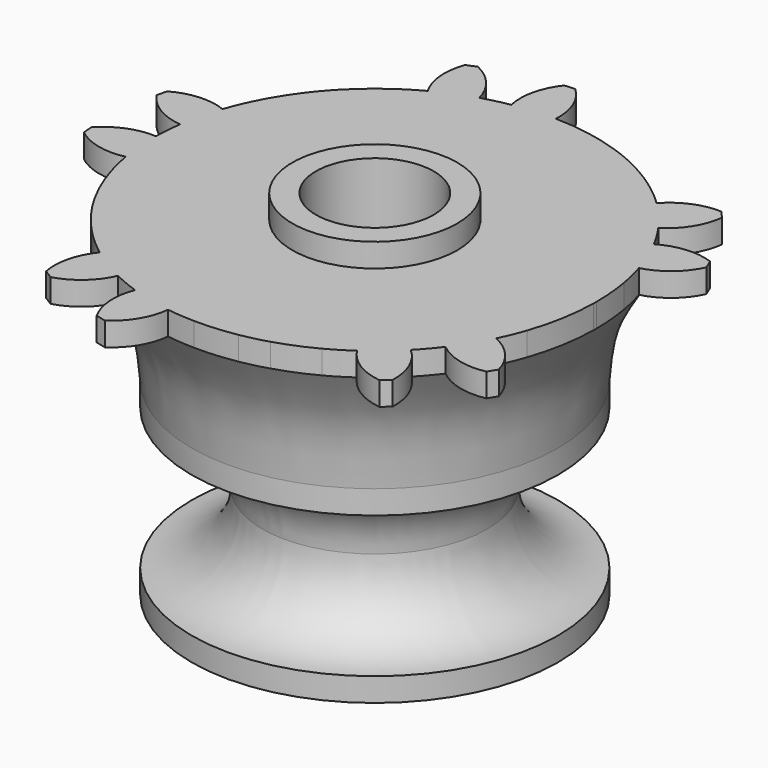
from build123d import *

# Parameters (mm, degrees)
F1_R      = 3.5
F1_R_2    = 2.5
F2_DEPTH  = 1
F3_DEPTH  = 2
F5_R      = 4.7747891135
F5_R_2    = 2.5
F6_DEPTH  = 6
F5_R_3    = 7.7747891135
F7_DEPTH  = 1
F8_DEPTH  = 6
F9_R      = 7.7747891135
F9_R_2    = 4.7747891135
F9_R_3    = 2.5
F10_DEPTH = 1


# Not quite as in the source:
# - a feature names something its author has since deleted; it is built from what else it names


with BuildPart() as f2:
    # F1 (on Top) → F2 (new body)
    with BuildSketch(Plane.XY):
        with BuildLine():
            ThreePointArc((-1.6229776334, 9.2680599554), (-0.7382287643, 9.3800858219), (0.1531520845, 9.4078443957))
            ThreePointArc((0.1531520845, 9.4078443957), (-0.0317997207, 10.5374998224), (-0.6817601701, 11.4797736507))
            Line((-0.6817601701, 11.4797736507), (-1.1224656787, 11.4450893749))
            ThreePointArc((-1.1224656787, 11.4450893749), (-1.6170199342, 10.4127402859), (-1.6229776334, 9.2680599554))
        make_face()
        with BuildLine():
            ThreePointArc((9.4078443957, -0.1531520845), (9.4087792756, -0.0765785786), (9.4090909091, 0))
            ThreePointArc((9.4090909091, 0), (9.3737668631, 0.8145468262), (9.2680599554, 1.6229776334))
            ThreePointArc((9.2680599554, 1.6229776334), (9.1491169783, 2.1965086508), (8.9947183137, 2.7615275108))
            ThreePointArc((8.9947183137, 2.7615275108), (8.6928665104, 3.6007032045), (8.3129211438, 4.4075314852))
            ThreePointArc((8.3129211438, 4.4075314852), (8.0225688191, 4.9162364953), (7.7011265332, 5.4058895526))
            ThreePointArc((7.7011265332, 5.4058895526), (7.1547288581, 6.1107157275), (6.5440556911, 6.7606454461))
            ThreePointArc((6.5440556911, 6.7606454461), (6.1107157275, 7.1547288581), (5.6536948308, 7.52108546))
            ThreePointArc((5.6536948308, 7.52108546), (4.9162364953, 8.0225688191), (4.1346124722, 8.4519803265))
            ThreePointArc((4.1346124722, 8.4519803265), (3.6007032045, 8.6928665104), (3.0528400867, 8.90006512))
            ThreePointArc((3.0528400867, 8.90006512), (2.1965086508, 9.1491169783), (1.320444577, 9.3159764842))
            ThreePointArc((1.320444577, 9.3159764842), (0.7382287643, 9.3800858219), (0.1531520845, 9.4078443957))
            ThreePointArc((0.1531520845, 9.4078443957), (-0.7382287643, 9.3800858219), (-1.6229776334, 9.2680599554))
            ThreePointArc((-1.6229776334, 9.2680599554), (-2.1965086508, 9.1491169783), (-2.7615275108, 8.9947183137))
            ThreePointArc((-2.7615275108, 8.9947183137), (-3.6007032045, 8.6928665104), (-4.4075314852, 8.3129211438))
            ThreePointArc((-4.4075314852, 8.3129211438), (-4.9162364953, 8.0225688191), (-5.4058895526, 7.7011265332))
            ThreePointArc((-5.4058895526, 7.7011265332), (-6.1107157275, 7.1547288581), (-6.7606454461, 6.5440556911))
            ThreePointArc((-6.7606454461, 6.5440556911), (-7.1547288581, 6.1107157275), (-7.52108546, 5.6536948308))
            ThreePointArc((-7.52108546, 5.6536948308), (-8.0225688191, 4.9162364953), (-8.4519803265, 4.1346124722))
            ThreePointArc((-8.4519803265, 4.1346124722), (-8.6928665104, 3.6007032045), (-8.90006512, 3.0528400867))
            ThreePointArc((-8.90006512, 3.0528400867), (-9.1491169783, 2.1965086508), (-9.3159764842, 1.320444577))
            ThreePointArc((-9.3159764842, 1.320444577), (-9.3800858219, 0.7382287643), (-9.4078443957, 0.1531520845))
            ThreePointArc((-9.4078443957, 0.1531520845), (-9.3800858219, -0.7382287643), (-9.2680599554, -1.6229776334))
            ThreePointArc((-9.2680599554, -1.6229776334), (-9.1491169783, -2.1965086508), (-8.9947183137, -2.7615275108))
            ThreePointArc((-8.9947183137, -2.7615275108), (-8.6928665104, -3.6007032045), (-8.3129211438, -4.4075314852))
            ThreePointArc((-8.3129211438, -4.4075314852), (-8.0225688191, -4.9162364953), (-7.7011265332, -5.4058895526))
            ThreePointArc((-7.7011265332, -5.4058895526), (-7.1547288581, -6.1107157275), (-6.5440556911, -6.7606454461))
            ThreePointArc((-6.5440556911, -6.7606454461), (-6.1107157275, -7.1547288581), (-5.6536948308, -7.52108546))
            ThreePointArc((-5.6536948308, -7.52108546), (-4.9162364953, -8.0225688191), (-4.1346124722, -8.4519803265))
            ThreePointArc((-4.1346124722, -8.4519803265), (-3.6007032045, -8.6928665104), (-3.0528400867, -8.90006512))
            ThreePointArc((-3.0528400867, -8.90006512), (-2.1965086508, -9.1491169783), (-1.320444577, -9.3159764842))
            ThreePointArc((-1.320444577, -9.3159764842), (-0.7382287643, -9.3800858219), (-0.1531520845, -9.4078443957))
            ThreePointArc((-0.1531520845, -9.4078443957), (0.7382287643, -9.3800858219), (1.6229776334, -9.2680599554))
            ThreePointArc((1.6229776334, -9.2680599554), (2.1965086508, -9.1491169783), (2.7615275108, -8.9947183137))
            ThreePointArc((2.7615275108, -8.9947183137), (3.6007032045, -8.6928665104), (4.4075314852, -8.3129211438))
            ThreePointArc((4.4075314852, -8.3129211438), (4.9162364953, -8.0225688191), (5.4058895526, -7.7011265332))
            ThreePointArc((5.4058895526, -7.7011265332), (6.1107157275, -7.1547288581), (6.7606454461, -6.5440556911))
            ThreePointArc((6.7606454461, -6.5440556911), (7.1547288581, -6.1107157275), (7.52108546, -5.6536948308))
            ThreePointArc((7.52108546, -5.6536948308), (8.0225688191, -4.9162364953), (8.4519803265, -4.1346124722))
            ThreePointArc((8.4519803265, -4.1346124722), (8.6928665104, -3.6007032045), (8.90006512, -3.0528400867))
            ThreePointArc((8.90006512, -3.0528400867), (9.1491169783, -2.1965086508), (9.3159764842, -1.320444577))
            ThreePointArc((9.3159764842, -1.320444577), (9.3800858219, -0.7382287643), (9.4078443957, -0.1531520845))
        make_face()
        Circle(F1_R, mode=Mode.SUBTRACT)
        with BuildLine():
            ThreePointArc((-4.4075314852, 8.3129211438), (-3.6007032045, 8.6928665104), (-2.7615275108, 8.9947183137))
            ThreePointArc((-2.7615275108, 8.9947183137), (-3.286509855, 10.0119312174), (-4.195837602, 10.7072380574))
            Line((-4.195837602, 10.7072380574), (-4.604255417, 10.5380658593))
            ThreePointArc((-4.604255417, 10.5380658593), (-4.7555910517, 9.4034178615), (-4.4075314852, 8.3129211438))
        make_face()
        with BuildLine():
            ThreePointArc((-9.3159764842, 1.320444577), (-9.1491169783, 2.1965086508), (-8.90006512, 3.0528400867))
            ThreePointArc((-8.90006512, 3.0528400867), (-10.0315845257, 3.2260231917), (-11.1285890147, 2.8990526973))
            Line((-11.1285890147, 2.8990526973), (-11.2317877999, 2.469198821))
            ThreePointArc((-11.2317877999, 2.469198821), (-10.4027911413, 1.679836361), (-9.3159764842, 1.320444577))
        make_face()
        with BuildLine():
            ThreePointArc((-9.2680599554, -1.6229776334), (-9.3800858219, -0.7382287643), (-9.4078443957, 0.1531520845))
            ThreePointArc((-9.4078443957, 0.1531520845), (-10.5374998224, -0.0317997207), (-11.4797736507, -0.6817601701))
            Line((-11.4797736507, -0.6817601701), (-11.4450893749, -1.1224656787))
            ThreePointArc((-11.4450893749, -1.1224656787), (-10.4127402859, -1.6170199342), (-9.2680599554, -1.6229776334))
        make_face()
        with BuildLine():
            ThreePointArc((-5.8191609361, -9.9190405786), (-4.812258569, -9.3745443193), (-4.1346124722, -8.4519803265))
            ThreePointArc((-4.1346124722, -8.4519803265), (-4.9162364953, -8.0225688191), (-5.6536948308, -7.52108546))
            ThreePointArc((-5.6536948308, -7.52108546), (-6.1680604771, -8.5437078414), (-6.1960860878, -9.6880605486))
            Line((-6.1960860878, -9.6880605486), (-5.8191609361, -9.9190405786))
        make_face()
        with BuildLine():
            ThreePointArc((-2.469198821, -11.2317877999), (-1.679836361, -10.4027911413), (-1.320444577, -9.3159764842))
            ThreePointArc((-1.320444577, -9.3159764842), (-2.1965086508, -9.1491169783), (-3.0528400867, -8.90006512))
            ThreePointArc((-3.0528400867, -8.90006512), (-3.2260231917, -10.0315845257), (-2.8990526973, -11.1285890147))
            Line((-2.8990526973, -11.1285890147), (-2.469198821, -11.2317877999))
        make_face()
        with BuildLine():
            ThreePointArc((7.6353485554, -8.5995030343), (7.428651783, -7.4736233793), (6.7606454461, -6.5440556911))
            ThreePointArc((6.7606454461, -6.5440556911), (6.1107157275, -7.1547288581), (5.4058895526, -7.7011265332))
            ThreePointArc((5.4058895526, -7.7011265332), (6.2195135061, -8.5063250277), (7.2991972152, -8.8866034014))
            Line((7.2991972152, -8.8866034014), (7.6353485554, -8.5995030343))
        make_face()
        with BuildLine():
            ThreePointArc((9.9190405786, -5.8191609361), (9.3745443193, -4.812258569), (8.4519803265, -4.1346124722))
            ThreePointArc((8.4519803265, -4.1346124722), (8.0225688191, -4.9162364953), (7.52108546, -5.6536948308))
            ThreePointArc((7.52108546, -5.6536948308), (8.5437078414, -6.1680604771), (9.6880605486, -6.1960860878))
            Line((9.6880605486, -6.1960860878), (9.9190405786, -5.8191609361))
        make_face()
        with BuildLine():
            ThreePointArc((8.3129211438, 4.4075314852), (8.6928665104, 3.6007032045), (8.9947183137, 2.7615275108))
            ThreePointArc((8.9947183137, 2.7615275108), (10.0119312174, 3.286509855), (10.7072380574, 4.195837602))
            Line((10.7072380574, 4.195837602), (10.5380658593, 4.604255417))
            ThreePointArc((10.5380658593, 4.604255417), (9.4034178615, 4.7555910517), (8.3129211438, 4.4075314852))
        make_face()
        with BuildLine():
            ThreePointArc((6.5440556911, 6.7606454461), (7.1547288581, 6.1107157275), (7.7011265332, 5.4058895526))
            ThreePointArc((7.7011265332, 5.4058895526), (8.5063250277, 6.2195135061), (8.8866034014, 7.2991972152))
            Line((8.8866034014, 7.2991972152), (8.5995030343, 7.6353485554))
            ThreePointArc((8.5995030343, 7.6353485554), (7.4736233793, 7.428651783), (6.5440556911, 6.7606454461))
        make_face()
        Circle(F1_R)
        Circle(F1_R_2, mode=Mode.SUBTRACT)
    extrude(amount=F2_DEPTH)

    # F1 (on Top) → F3 (join)
    with BuildSketch(Plane.XY):
        Circle(F1_R)
        Circle(F1_R_2, mode=Mode.SUBTRACT)
    extrude(amount=F3_DEPTH)

    # F5 (on offset) → F6 (join, through all)
    with BuildSketch(Plane.XY.offset(-6)):
        Circle(F5_R)
        Circle(F5_R_2, mode=Mode.SUBTRACT)
    extrude(amount=F6_DEPTH)

    # F5 (on offset) → F7 (join)
    with BuildSketch(Plane.XY.offset(-6)):
        Circle(F5_R_3)
        Circle(F5_R, mode=Mode.SUBTRACT)
    extrude(amount=F7_DEPTH)

    # F5 (on offset) → F8 (join)
    with BuildSketch(Plane.XY.offset(-6)):
        Circle(F5_R)
        Circle(F5_R_2, mode=Mode.SUBTRACT)
    extrude(amount=-F8_DEPTH)

    # F9 (on face) → F10 (join)
    with BuildSketch(Plane(origin=(0, 0, -12), x_dir=(1, 0, 0), z_dir=(0, 0, -1))):
        Circle(F9_R)
        Circle(F9_R_2, mode=Mode.SUBTRACT)
        Circle(F9_R_2)
        Circle(F9_R_3, mode=Mode.SUBTRACT)
    extrude(amount=F10_DEPTH)

    # F11 (on Front) → F12 (revolve)
    with BuildSketch(Plane.XZ):
        with BuildLine():
            Line((7.7747891135, -6), (4.7747891135, -6))
            Line((4.7747891135, -6), (4.7747891135, -9))
            ThreePointArc((4.7747891135, -9), (5.6534687699, -6.8786796564), (7.7747891135, -6))
        make_face()
        with BuildLine():
            ThreePointArc((7.7747891135, -12), (5.6534687699, -11.1213203436), (4.7747891135, -9))
            Line((4.7747891135, -9), (4.7747891135, -12))
            Line((4.7747891135, -12), (7.7747891135, -12))
        make_face()
        with BuildLine():
            add(Edge.make_bspline(
                [(7.7747891135, -5), (7.8420486188, -4.1163054386), (7.9641288698, -2.3547490655), (8.9230440814, -0.790182696), (9.4090909091, 0)],
                knots=[0, 0, 0, 0, 0.4946853103, 1, 1, 1, 1], degree=3))
            Line((9.4090909091, 0), (4.7747891135, 0))
            Line((4.7747891135, 0), (4.7747891135, -5))
            Line((4.7747891135, -5), (7.7747891135, -5))
        make_face()
    revolve(axis=Axis((0, 0, -9.1715450399), (0, 0, -1)))


solid = f2.part
